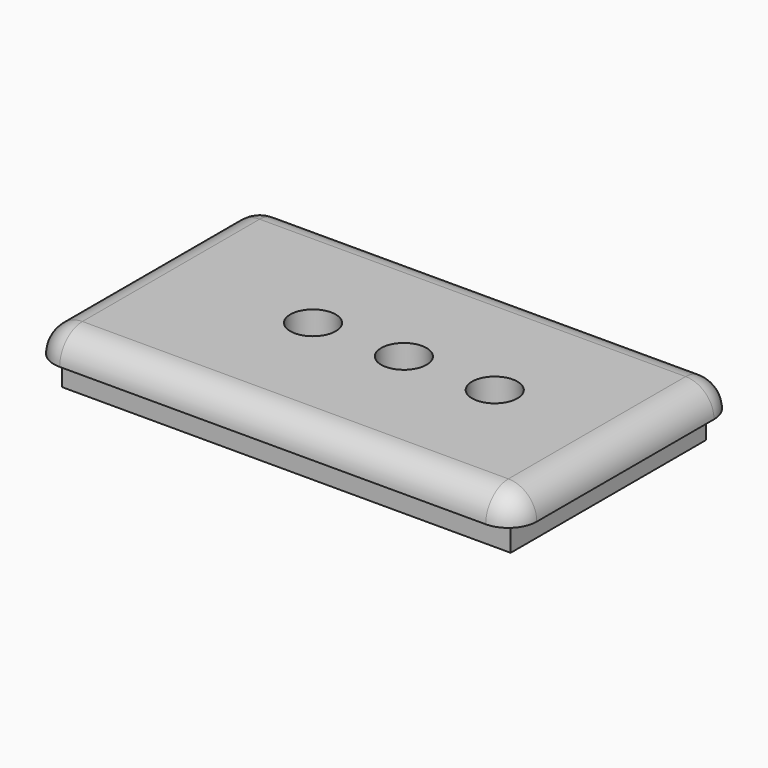
from build123d import *

# Parameters (mm, degrees)
F0_W     = 53.975
F0_H     = 31.115
F1_DEPTH = 3.175
F2_R     = 3.17499
F3_W     = 50.165
F3_H     = 27.305
F3_W_2   = 47.625
F3_H_2   = 24.765
F4_DEPTH = 3.175
F6_D     = 5.08


# Not quite as in the source:
# - a fillet or chamfer is up to 0.001 mm smaller than in the source, because OpenCascade refuses the exact size


with BuildPart() as f1:
    # F0 (on Top) → F1 (new body)
    with BuildSketch(Plane.XY):
        Rectangle(F0_W, F0_H)
    extrude(amount=F1_DEPTH)

    # F2 (radius 3.175 in the source; OpenCascade refuses exactly that, so slightly less here)
    f2_edges = [f1.edges().sort_by_distance(p)[0] for p in [
        (0, -15.5575, 3.175),
        (-26.9875, 0, 3.175),
        (0, 15.5575, 3.175),
        (26.9875, 0, 3.175),
        (26.9875, -15.5575, 1.5875),
        (26.9875, 15.5575, 1.5875),
        (-26.9875, 15.5575, 1.5875),
        (-26.9875, -15.5575, 1.5875),
    ]]
    fillet(f2_edges, radius=F2_R)

    # F3 (on face) → F4 (join)
    with BuildSketch(Plane(origin=(0, 0, 0), x_dir=(1, 0, 0), z_dir=(0, 0, -1))):
        Rectangle(F3_W, F3_H)
        Rectangle(F3_W_2, F3_H_2, mode=Mode.SUBTRACT)
    extrude(amount=F4_DEPTH)

    # F6 (through all)
    with Locations(Plane.XY.offset(3.175)):
        with Locations((-7.9375, 0), (2.2225, 0), (12.3825, 0)):
            Hole(F6_D / 2)


solid = f1.part
